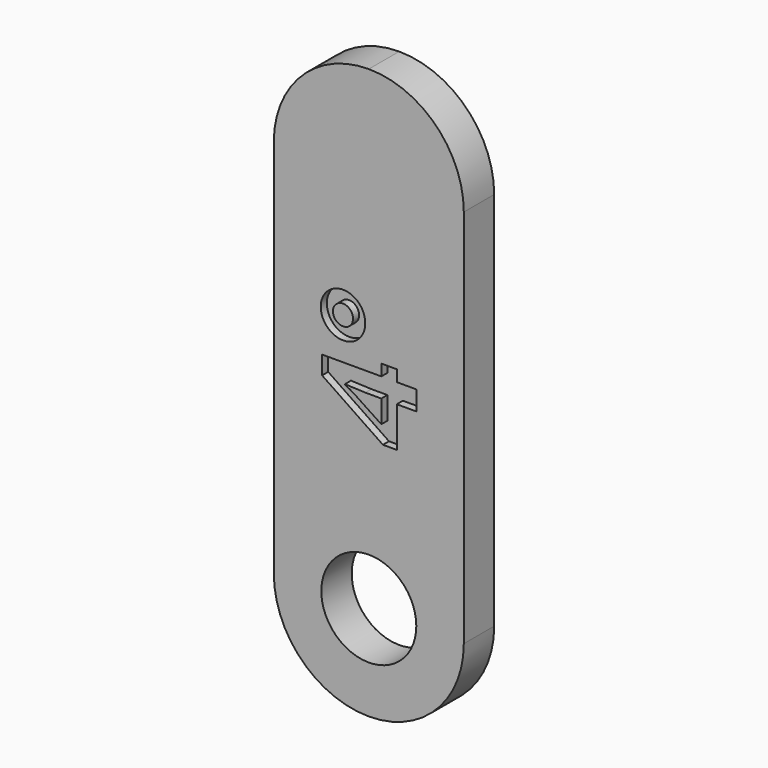
from build123d import *

# Parameters (mm, degrees)
F0_W         = 12.7
F0_H         = 38.1
F0_R         = 3.175
F1_DEPTH     = 2.54
F2_R         = 6.34999
F3_TEXT_SIZE = 8.8194444444
F4_DEPTH     = 0.508


# Not quite as in the source:
# - a fillet or chamfer is up to 0.001 mm smaller than in the source, because OpenCascade refuses the exact size
# - Text() gives the source's letters only with a copy of the font that has no kerning and outlines rounded to 1/6400 em; it was checked with that copy


with BuildPart() as f1:
    # F0 (on Front) → F1 (new body)
    with BuildSketch(Plane.XZ):
        with Locations((6.35, 19.05)):
            Rectangle(F0_W, F0_H)
        with Locations((6.35, 6.35)):
            Circle(F0_R, mode=Mode.SUBTRACT)
    extrude(amount=F1_DEPTH)

    # F2 (radius 6.35 in the source; OpenCascade refuses exactly that, so slightly less here)
    f2_edges = [f1.edges().sort_by_distance(p)[0] for p in [
        (12.7, -1.27, 0),
        (0, -1.27, 0),
        (12.7, -1.27, 38.1),
        (0, -1.27, 38.1),
    ]]
    fillet(f2_edges, radius=F2_R)

    # F3 (on face) → F4 (cut)
    with BuildSketch(Plane.XZ.offset(2.54)):
        with Locations(Location((9.525, 16.1464735243), (0, 0, 90))):
            Text('4°', F3_TEXT_SIZE, font='Open Sans', font_style=FontStyle.BOLD, text_align=(TextAlign.LEFT, TextAlign.BOTTOM))
    extrude(amount=-F4_DEPTH, mode=Mode.SUBTRACT)


solid = f1.part
